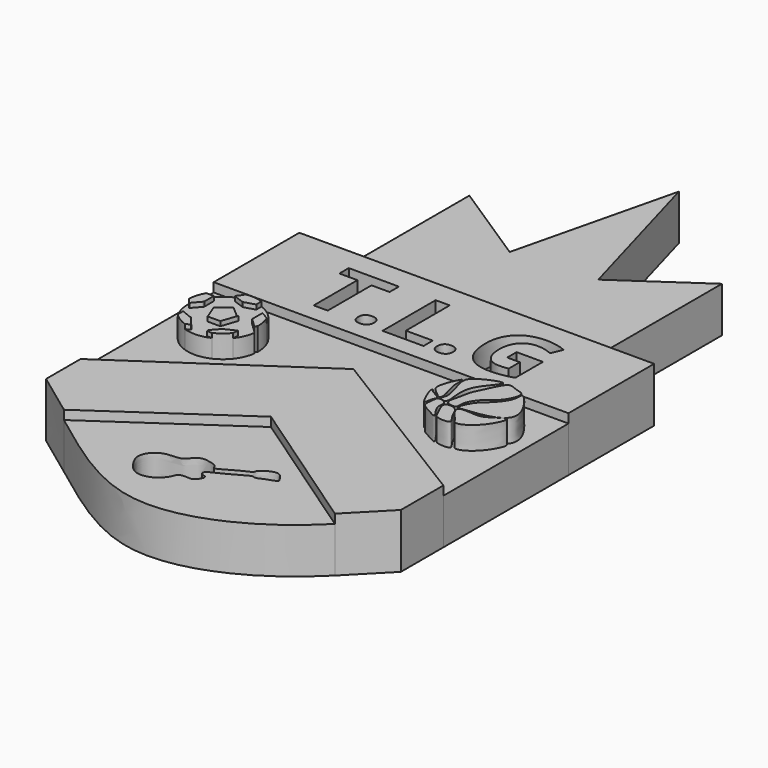
from build123d import *

# Parameters (mm, degrees)
F1_DEPTH     = 6.35
F3_DEPTH     = 7.62
F4_TEXT_SIZE = 13.0019900906
F5_DEPTH     = 3.175
F6_DEPTH     = 3.175
F8_DEPTH     = 3.175
F9_DEPTH     = 2.54
F10_DEPTH    = 3.175
F12_DEPTH    = 3.175


# Not quite as in the source:
# - Text() gives the source's letters only with a copy of the font that has no kerning and outlines rounded to 1/6400 em; it was checked with that copy


with BuildPart() as f1:
    # F0 (on Top) → F1 (new body)
    with BuildSketch(Plane.XY):
        Polygon((-14.5788859001, 11.2244244665), (-64.1806870699, 11.2244244665), (-64.1806870699, -12.0365046459), (-39.4293889403, 4.7148435568), (-14.5788859001, -10.6420014073), align=None)
    extrude(amount=F1_DEPTH)

    # F4 (on face) → F5 (cut)
    with BuildSketch(Plane.XY.offset(7.62)):
        with Locations((-55.0058893859, 13.7539170682)):
            Text('T.L.G', F4_TEXT_SIZE, font='Open Sans', font_style=FontStyle.BOLD, text_align=(TextAlign.LEFT, TextAlign.BOTTOM))
    extrude(amount=F5_DEPTH, mode=Mode.SUBTRACT)

    # F7 (on face) → F8 (join)
    with BuildSketch(Plane.XY.offset(6.35)):
        with BuildLine():
            Line((-54.9722793177, 7.2115763099), (-54.9722793177, 8.063433158))
            ThreePointArc((-54.9722793177, 8.063433158), (-56.1346983589, 8.3186356437), (-57.3244372717, 8.2891796507))
            Line((-57.3244372717, 8.2891796507), (-57.6540782349, 7.7934470537))
            Line((-57.6540782349, 7.7934470537), (-58.0486051039, 7.2805625896))
            Line((-58.0486051039, 7.2805625896), (-58.0227002501, 7.231569849))
            Line((-58.0227002501, 7.231569849), (-56.4840473235, 6.6792317666))
            Line((-56.4840473235, 6.6792317666), (-56.4051419497, 6.7186844535))
            Line((-56.4051419497, 6.7186844535), (-54.9453943968, 7.1526640095))
            Line((-54.9453943968, 7.1526640095), (-54.9722793177, 7.2115763099))
        make_face()
        Polygon((-54.9453943968, 3.720282577), (-56.4840473235, 5.0616730005), (-58.1280679653, 3.647049937), (-57.3520064354, 1.6292912187), (-55.6160882115, 1.6292912187), (-55.5766373873, 1.6292912187), (-54.8270344734, 3.838640172), align=None)
        with BuildLine():
            ThreePointArc((-51.6572857624, 3.2389379273), (-51.6555929238, 3.3136850455), (-51.6550286015, 3.3884492008))
            ThreePointArc((-51.6550286015, 3.3884492008), (-51.7530661236, 4.3690189651), (-52.0432975412, 5.3107695385))
            Line((-52.0432975412, 5.3107695385), (-52.4993278086, 5.6140101515))
            Line((-52.4993278086, 5.6140101515), (-53.2489307225, 6.0085370205))
            Line((-53.2489307225, 6.0085370205), (-53.1700253487, 5.8901789598))
            Line((-53.1700253487, 5.8901789598), (-53.1700253487, 4.1937143542))
            Line((-53.1700253487, 4.1937143542), (-51.8781379587, 2.9530644734))
            Line((-51.8781379587, 2.9530644734), (-51.6572857624, 3.2389379273))
        make_face()
        with BuildLine():
            Line((-59.8375238341, 5.8388877454), (-60.9120507589, 5.8388877454))
            ThreePointArc((-60.9120507589, 5.8388877454), (-61.3602901488, 4.7831258584), (-61.553662218, 3.6525689357))
            Line((-61.553662218, 3.6525689357), (-61.4945366979, 3.5624715965))
            Line((-61.4945366979, 3.5624715965), (-60.9027445316, 2.8523236979))
            Line((-60.9027445316, 2.8523236979), (-60.9027445316, 2.8917763848))
            Line((-60.9027445316, 2.8917763848), (-59.9164292216, 4.0359036066))
            Line((-59.9164292216, 4.0359036066), (-59.8375238341, 4.1542616673))
            Line((-59.8375238341, 4.1542616673), (-59.8375238341, 5.8388877454))
        make_face()
        with BuildLine():
            ThreePointArc((-60.2103142537, -0.0105238415), (-59.2821338814, -0.7803559908), (-58.1954247645, -1.3030639752))
            Line((-58.1954247645, -1.3030639752), (-57.5477184431, -1.0133980707))
            Line((-57.5477184431, -1.0133980707), (-57.5887225568, -0.9351319168))
            Line((-57.5887225568, -0.9351319168), (-58.6539432406, 0.3273533075))
            Line((-58.6539432406, 0.3273533075), (-58.7709804456, 0.3273903499))
            Line((-58.7709804456, 0.3273903499), (-60.2103142537, 0.9191830476))
            Line((-60.2103142537, 0.9191830476), (-60.2103142537, -0.0105238415))
        make_face()
        with BuildLine():
            ThreePointArc((-54.5531226461, -1.1180623052), (-53.5600965179, -0.5156142275), (-52.7346804856, 0.3015350558))
            Line((-52.7346804856, 0.3015350558), (-52.6571385562, 1.0769538349))
            Line((-52.6571385562, 1.0769538349), (-54.2352460325, 0.3273533075))
            Line((-54.2352460325, 0.3273533075), (-55.261015892, -0.8167739143))
            Line((-55.261015892, -0.8167739143), (-55.2610189305, -1.1180623052))
            Line((-55.2610189305, -1.1180623052), (-54.5531226461, -1.1180623052))
        make_face()
    extrude(amount=F8_DEPTH)

    # F7 (on face) → F9 (join)
    with BuildSketch(Plane.XY.offset(6.35)):
        with BuildLine():
            Line((-52.4993278086, 5.6140101515), (-52.0432975412, 5.3107695385))
            ThreePointArc((-52.0432975412, 5.3107695385), (-53.2159980205, 6.9975819985), (-54.9722793177, 8.063433158))
            Line((-54.9722793177, 8.063433158), (-54.9722793177, 7.2115763099))
            Line((-54.9722793177, 7.2115763099), (-54.9453943968, 7.1526640095))
            Line((-54.9453943968, 7.1526640095), (-56.4051419497, 6.7186844535))
            Line((-56.4051419497, 6.7186844535), (-56.4840473235, 6.6792317666))
            Line((-56.4840473235, 6.6792317666), (-58.0227002501, 7.231569849))
            Line((-58.0227002501, 7.231569849), (-58.0486051039, 7.2805625896))
            Line((-58.0486051039, 7.2805625896), (-57.6540782349, 7.7934470537))
            Line((-57.6540782349, 7.7934470537), (-57.3244372717, 8.2891796507))
            ThreePointArc((-57.3244372717, 8.2891796507), (-59.4012478453, 7.4783959034), (-60.9120507589, 5.8388877454))
            Line((-60.9120507589, 5.8388877454), (-59.8375238341, 5.8388877454))
            Line((-59.8375238341, 5.8388877454), (-59.8375238341, 4.1542616673))
            Line((-59.8375238341, 4.1542616673), (-59.9164292216, 4.0359036066))
            Line((-59.9164292216, 4.0359036066), (-60.9027445316, 2.8917763848))
            Line((-60.9027445316, 2.8917763848), (-60.9027445316, 2.8523236979))
            Line((-60.9027445316, 2.8523236979), (-61.4945366979, 3.5624715965))
            Line((-61.4945366979, 3.5624715965), (-61.553662218, 3.6525689357))
            ThreePointArc((-61.553662218, 3.6525689357), (-61.2578859336, 1.6831714367), (-60.2103142537, -0.0105238415))
            Line((-60.2103142537, -0.0105238415), (-60.2103142537, 0.9191830476))
            Line((-60.2103142537, 0.9191830476), (-58.7709804456, 0.3273903499))
            Line((-58.7709804456, 0.3273903499), (-58.6539432406, 0.3273533075))
            Line((-58.6539432406, 0.3273533075), (-57.5887225568, -0.9351319168))
            Line((-57.5887225568, -0.9351319168), (-57.5477184431, -1.0133980707))
            Line((-57.5477184431, -1.0133980707), (-58.1954247645, -1.3030639752))
            ThreePointArc((-58.1954247645, -1.3030639752), (-56.3566257652, -1.5580147578), (-54.5531226461, -1.1180623052))
            Line((-54.5531226461, -1.1180623052), (-55.2610189305, -1.1180623052))
            Line((-55.2610189305, -1.1180623052), (-55.261015892, -0.8167739143))
            Line((-55.261015892, -0.8167739143), (-54.2352460325, 0.3273533075))
            Line((-54.2352460325, 0.3273533075), (-52.6571385562, 1.0769538349))
            Line((-52.6571385562, 1.0769538349), (-52.7346804856, 0.3015350558))
            ThreePointArc((-52.7346804856, 0.3015350558), (-52.0431181214, 1.4665549532), (-51.6931180042, 2.7753825901))
            Line((-51.6931180042, 2.7753825901), (-51.8781379587, 2.9530644734))
            Line((-51.8781379587, 2.9530644734), (-53.1700253487, 4.1937143542))
            Line((-53.1700253487, 4.1937143542), (-53.1700253487, 5.8901789598))
            Line((-53.1700253487, 5.8901789598), (-53.2489307225, 6.0085370205))
            Line((-53.2489307225, 6.0085370205), (-52.4993278086, 5.6140101515))
        make_face()
        Polygon((-58.1280679653, 3.647049937), (-56.4840473235, 5.0616730005), (-54.9453943968, 3.720282577), (-54.8270344734, 3.838640172), (-55.5766373873, 1.6292912187), (-55.6160882115, 1.6292912187), (-57.3520064354, 1.6292912187), align=None, mode=Mode.SUBTRACT)
    extrude(amount=F9_DEPTH)


with BuildPart() as f1b:
    # F0 (on Top) → F1, piece 2 (new body)
    with BuildSketch(Plane.XY):
        with BuildLine():
            Line((-39.4293889403, -9.7100831237), (-58.1129881465, -22.5383668142))
            add(Edge.make_bspline(
                [(-58.1129881465, -22.5383668142), (-51.6041701361, -27.4298691774), (-40.7768113234, -35.5562156994), (-26.4086529743, -29.4268878898), (-21.069979989, -24.6283628223), (-19.6609603516, -23.2431711295)],
                knots=[0.0914388924, 0.0914388924, 0.0914388924, 0.0914388924, 0.4026792113, 0.7190173036, 0.8439557876, 0.8439557876, 0.8439557876, 0.8439557876], degree=3))
            Line((-19.6609603516, -23.2431711295), (-39.4293889403, -9.7100831237))
        make_face()
    extrude(amount=F1_DEPTH)

    # F11 (on face) → F12 (cut)
    with BuildSketch(Plane.XY.offset(6.35)):
        with BuildLine():
            add(Edge.make_bspline(
                [(-39.6092943847, -20.2816836536), (-39.9787013912, -20.2032415358), (-40.6095365727, -20.0671132852), (-41.5650695108, -20.715600161), (-41.9382638002, -21.4005518257), (-42.6223838474, -21.7366043809), (-43.7793923029, -21.7320661055), (-45.0038375213, -21.9481501705), (-46.103436005, -22.7881190245), (-46.6664233936, -24.2612544081), (-45.8951348827, -25.7374611984), (-44.7520992773, -27.2891773412), (-42.9235035722, -27.5571003667), (-41.2583010505, -26.6655893757), (-40.5423333626, -25.4840664669), (-40.3629851855, -24.6811028122), (-39.0404800063, -24.6866250406), (-38.2009304906, -24.7793118248), (-37.2865756943, -23.2160512599), (-38.4420072291, -23.25658414), (-38.6100637674, -22.4460098243), (-37.2473937849, -21.9800136549), (-34.1010097641, -20.1466160398), (-33.7231439394, -19.9861618912), (-33.2223238288, -20.2879889522), (-32.2022801847, -19.6194761769), (-30.5295871592, -19.2710510174), (-31.1374592405, -18.5543296466), (-31.9615568407, -17.1974263449), (-34.3091596328, -18.6887967691), (-34.1353943562, -19.281929173), (-35.3803885686, -19.6109295765), (-38.0333084266, -21.3648709815), (-38.3255739116, -21.0871262618), (-38.4599904183, -20.5237302918), (-39.2163351135, -20.3651270017), (-39.6092943847, -20.2816836536)],
                knots=[0, 0, 0, 0, 0.027814881, 0.0563195996, 0.0805298145, 0.1036731277, 0.1333702249, 0.164282128, 0.1962589171, 0.229336563, 0.2644169784, 0.302262324, 0.3382503556, 0.3757277332, 0.4078764441, 0.4307877453, 0.4605320126, 0.4865810031, 0.5174388511, 0.5410936237, 0.560779126, 0.5933920103, 0.6467427869, 0.6634121617, 0.6815563263, 0.7126818691, 0.7454367308, 0.7669961919, 0.7989729459, 0.840661547, 0.8583114847, 0.8887823938, 0.9378210581, 0.9511829283, 0.970411727, 1, 1, 1, 1], degree=3))
        make_face()
    extrude(amount=-F12_DEPTH, mode=Mode.SUBTRACT)


with BuildPart() as f1c:
    # F0 (on Top) → F1, piece 3 (new body)
    with BuildSketch(Plane.XY):
        Polygon((-56.6977337003, 46.5509048615), (-56.6977337003, 26.1903237551), (-22.1364350356, 26.1903237551), (-22.1364350356, 47.4879480898), (-33.2914949005, 39.8288096684), (-39.4293889403, 61.5904293954), (-44.9334824718, 38.8904650835), align=None)
    extrude(amount=F1_DEPTH)


with BuildPart() as f3:
    # F0 (on Top) → F3 (new body)
    with BuildSketch(Plane.XY):
        Polygon((-56.6977337003, 26.1903237551), (-64.1806870699, 26.1903237551), (-64.1806870699, 11.2244244665), (-14.5788859001, 11.2244244665), (-14.5788859001, 26.1903237551), (-22.1364350356, 26.1903237551), align=None)
    extrude(amount=F3_DEPTH)

    # F4 (on face) → F6 (cut)
    with BuildSketch(Plane.XY.offset(7.62)):
        with Locations((-55.0058893859, 13.7539170682)):
            Text('T.L.G', F4_TEXT_SIZE, font='Open Sans', font_style=FontStyle.BOLD, text_align=(TextAlign.LEFT, TextAlign.BOTTOM))
    extrude(amount=-F6_DEPTH, mode=Mode.SUBTRACT)


with BuildPart() as f3b:
    # F0 (on Top) → F3, piece 2 (new body)
    with BuildSketch(Plane.XY):
        with BuildLine():
            Line((-39.4293889403, 4.7148435568), (-64.1806870699, -12.0365046459))
            Line((-64.1806870699, -12.0365046459), (-64.1806870699, -18.0648540245))
            add(Edge.make_bspline(
                [(-64.1806870699, -18.0648540245), (-62.0357416156, -19.5898871636), (-60.0252054074, -21.1012986344), (-58.1129881465, -22.5383668142)],
                knots=[0, 0, 0, 0, 0.0914388924, 0.0914388924, 0.0914388924, 0.0914388924], degree=3))
            Line((-58.1129881465, -22.5383668142), (-39.4293889403, -9.7100831237))
            Line((-39.4293889403, -9.7100831237), (-19.6609603516, -23.2431711295))
            add(Edge.make_bspline(
                [(-19.6609603516, -23.2431711295), (-17.9011394173, -21.513110544), (-16.3012369902, -19.7415763844), (-14.5788859001, -18.0648540245)],
                knots=[0.8439557876, 0.8439557876, 0.8439557876, 0.8439557876, 1, 1, 1, 1], degree=3))
            Line((-14.5788859001, -18.0648540245), (-14.5788859001, -10.6420014073))
            Line((-14.5788859001, -10.6420014073), (-39.4293889403, 4.7148435568))
        make_face()
    extrude(amount=F3_DEPTH)


with BuildPart() as f10:
    # F2 (on face) → F10 (new body)
    with BuildSketch(Plane.XY.offset(6.35)):
        with BuildLine():
            add(Edge.make_bspline(
                [(-22.3381277174, 9.4839343801), (-22.6403459871, 9.7312503516), (-26.15306833, 8.3014323162), (-26.1211835909, 6.5365833323), (-24.868463545, 3.3263104273), (-25.7169725821, 2.4861385653), (-24.1004826043, 1.7875739532), (-24.8019808117, 4.7476702348), (-24.2298518823, 7.1599000177), (-22.0791975146, 9.2720425752), (-22.3381277174, 9.4839343801)],
                knots=[0, 0, 0, 0, 0.1602097698, 0.2744410611, 0.4297722771, 0.5065686388, 0.5848602928, 0.7118486845, 0.8627377881, 1, 1, 1, 1], degree=3))
        make_face()
    extrude(amount=F10_DEPTH)


with BuildPart() as f10b:
    # F2 (on face) → F10, piece 2 (new body)
    with BuildSketch(Plane.XY.offset(6.35)):
        with BuildLine():
            add(Edge.make_bspline(
                [(-20.2133208513, 9.1664344072), (-20.6787451581, 9.3260038763), (-21.7410364909, 10.0979079014), (-22.8606364183, 7.060755168), (-23.7980614616, 5.6077840365), (-23.994350647, 3.6469853248), (-24.6266667674, 1.9700347275), (-22.5570899146, 1.6510712517), (-22.9642646953, 2.9356491733), (-21.7828679317, 5.081395851), (-19.5970025083, 6.2058963375), (-18.7054748685, 8.9967877923), (-19.7813384586, 9.0183304083), (-20.2133208513, 9.1664344072)],
                knots=[0, 0, 0, 0, 0.0795688858, 0.1913521005, 0.2866596603, 0.3834852999, 0.4655403256, 0.5431906503, 0.6082617659, 0.7126594458, 0.8243703251, 0.9261483399, 1, 1, 1, 1], degree=3))
        make_face()
    extrude(amount=F10_DEPTH)


with BuildPart() as f10c:
    # F2 (on face) → F10, piece 3 (new body)
    with BuildSketch(Plane.XY.offset(6.35)):
        with BuildLine():
            add(Edge.make_bspline(
                [(-18.8212059438, 8.4581654519), (-19.0070189305, 8.4258318729), (-18.6986089259, 6.9579464815), (-20.9135432611, 4.687655318), (-21.9572192628, 3.8959858631), (-22.9458478623, 1.6857991302), (-21.6866435241, 1.9936975585), (-19.2353013584, 2.0828209475), (-16.1027537635, 3.2548907156), (-16.4425817033, 5.9796450085), (-18.5204854365, 8.5104942501), (-18.8212059438, 8.4581654519)],
                knots=[0, 0, 0, 0, 0.0841946021, 0.2197568457, 0.3174826143, 0.4200315833, 0.4849886246, 0.6107170354, 0.7418743595, 0.8637391071, 1, 1, 1, 1], degree=3))
        make_face()
    extrude(amount=F10_DEPTH)


with BuildPart() as f10d:
    # F2 (on face) → F10, piece 4 (new body)
    with BuildSketch(Plane.XY.offset(6.35)):
        with BuildLine():
            add(Edge.make_bspline(
                [(-22.3381277174, 1.6441266052), (-22.0655906169, 1.9840001866), (-19.7550812828, 1.5571664137), (-18.5482539331, 2.0353127379), (-15.8749842673, 4.0779657614), (-17.7289459446, -0.0789688088), (-20.6099906945, -1.5586945132), (-20.9781001275, -0.4435148798), (-21.8471541344, 0.2228800877), (-22.5467458136, 1.38396467), (-22.3381277174, 1.6441266052)],
                knots=[0, 0, 0, 0, 0.1409371866, 0.2628688647, 0.3892674066, 0.5507402623, 0.7091139106, 0.7889088986, 0.8921172659, 1, 1, 1, 1], degree=3))
        make_face()
    extrude(amount=F10_DEPTH)


with BuildPart() as f10e:
    # F2 (on face) → F10, piece 5 (new body)
    with BuildSketch(Plane.XY.offset(6.35)):
        with BuildLine():
            add(Edge.make_bspline(
                [(-24.1210125387, 1.4975882368), (-24.3454889433, 1.0885757735), (-23.3383441576, -0.519984716), (-23.2306141185, -1.4627201909), (-20.4511683913, -1.5607358202), (-21.9734810782, -0.1779020509), (-22.3434818311, 1.7852269299), (-23.939485654, 1.8283435266), (-24.1210125387, 1.4975882368)],
                knots=[0, 0, 0, 0, 0.1922353713, 0.3274498981, 0.5052994982, 0.6529860043, 0.8445454072, 1, 1, 1, 1], degree=3))
        make_face()
    extrude(amount=F10_DEPTH)


with BuildPart() as f10f:
    # F2 (on face) → F10, piece 6 (new body)
    with BuildSketch(Plane.XY.offset(6.35)):
        with BuildLine():
            add(Edge.make_bspline(
                [(-25.537552312, 2.2302805446), (-25.7570178169, 2.1373048441), (-25.7325030733, 1.446952863), (-26.0677241402, 0.1480544144), (-24.9219521715, -0.4964252327), (-22.5508877802, -1.845968262), (-24.824203089, 0.5547512377), (-24.0078759967, 1.9189682407), (-25.2705121617, 2.3434110571), (-25.537552312, 2.2302805446)],
                knots=[0, 0, 0, 0, 0.1095724071, 0.2460244483, 0.3919415845, 0.5472864036, 0.7231839156, 0.866675029, 1, 1, 1, 1], degree=3))
        make_face()
    extrude(amount=F10_DEPTH)


with BuildPart() as f10g:
    # F2 (on face) → F10, piece 7 (new body)
    with BuildSketch(Plane.XY.offset(6.35)):
        with BuildLine():
            add(Edge.make_bspline(
                [(-27.4181291461, 3.3781651873), (-27.5233258284, 3.1203784065), (-26.8829474939, 1.54307483), (-26.1089252239, 0.2167874191), (-26.1261369658, 1.6797912135), (-25.4106712723, 2.4116569848), (-27.223963722, 3.0658664315), (-27.2281934669, 3.4997467106), (-27.388863119, 3.4498822297), (-27.4181291461, 3.3781651873)],
                knots=[0, 0, 0, 0, 0.2179330955, 0.3741879639, 0.5251993821, 0.6599610309, 0.8530149682, 0.9393703704, 1, 1, 1, 1], degree=3))
        make_face()
    extrude(amount=F10_DEPTH)


with BuildPart() as f10h:
    # F2 (on face) → F10, piece 8 (new body)
    with BuildSketch(Plane.XY.offset(6.35)):
        with BuildLine():
            add(Edge.make_bspline(
                [(-25.6676729769, 2.5971706491), (-25.8897838153, 2.5151853008), (-26.8942863412, 3.4706843257), (-27.5908830964, 4.0169316753), (-27.1448249564, 5.9187892116), (-26.0713429056, 7.989770409), (-26.3385063597, 5.5599874191), (-25.6583843497, 4.0877353512), (-25.4596195189, 2.6739671501), (-25.6676729769, 2.5971706491)],
                knots=[0, 0, 0, 0, 0.1393046045, 0.2509379196, 0.4167774681, 0.5580584925, 0.6996161524, 0.8695119748, 1, 1, 1, 1], degree=3))
        make_face()
    extrude(amount=F10_DEPTH)


solid = Compound([f1.part, f1b.part, f1c.part, f3.part, f3b.part, f10.part, f10b.part, f10c.part, f10d.part, f10e.part, f10f.part, f10g.part, f10h.part])
